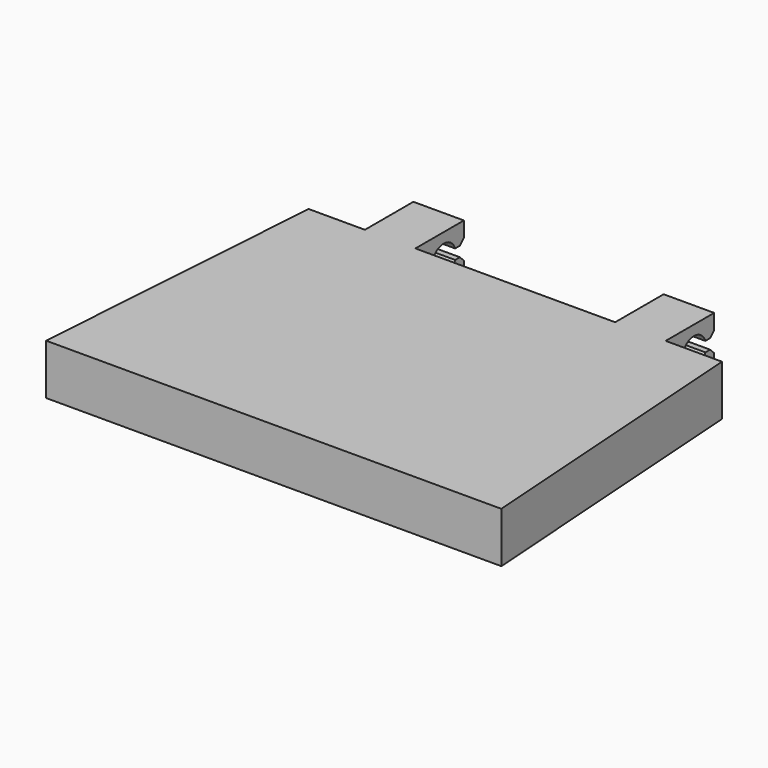
from build123d import *

# Parameters (mm, degrees)
F1_DEPTH = 5
F4_DEPTH = 45.5
F5_SIZE  = 0.5


with BuildPart() as f1:
    # F0 (on Top) → F1 (new body)
    with BuildSketch(Plane.XY):
        Polygon((-14.8876575074, 87.1), (-20.4571957112, 87.1), (-22.5358384183, 57.2079033579), (22.5358384183, 57.2079033579), (20.4571957112, 87.1), (14.8876575074, 87.1), (14.8876575074, 93.1), (9.8876575074, 93.1), (9.8876575074, 87.1), (-9.8876575074, 87.1), (-9.8876575074, 93.1), (-14.8876575074, 93.1), align=None)
    extrude(amount=F1_DEPTH)

    # F3 (on offset) → F4 (cut)
    with BuildSketch(Plane.YZ.offset(24.8876575074)):
        with BuildLine():
            Line((95.6, 3), (92.0142135624, 3))
            ThreePointArc((92.0142135624, 3), (90.4708684127, 3.9944313411), (89.1209800542, 2.75))
            Line((89.1209800542, 2.75), (88.1, 2.75))
            Line((88.1, 2.75), (88.1, 2.25))
            Line((88.1, 2.25), (89.1209800542, 2.25))
            ThreePointArc((89.1209800542, 2.25), (90.4708684127, 1.0055686589), (92.0142135624, 2))
            Line((92.0142135624, 2), (95.6, 2))
            Line((95.6, 2), (95.6, 3))
        make_face()
    extrude(amount=-F4_DEPTH, mode=Mode.SUBTRACT)

    # F5
    f5_edges = [f1.edges().sort_by_distance(p)[0] for p in [
        (-12.387658, 93.1, 3),
        (-12.387658, 93.1, 2),
        (12.387658, 93.1, 3),
        (12.387658, 93.1, 2),
    ]]
    chamfer(f5_edges, length=F5_SIZE)


solid = f1.part
